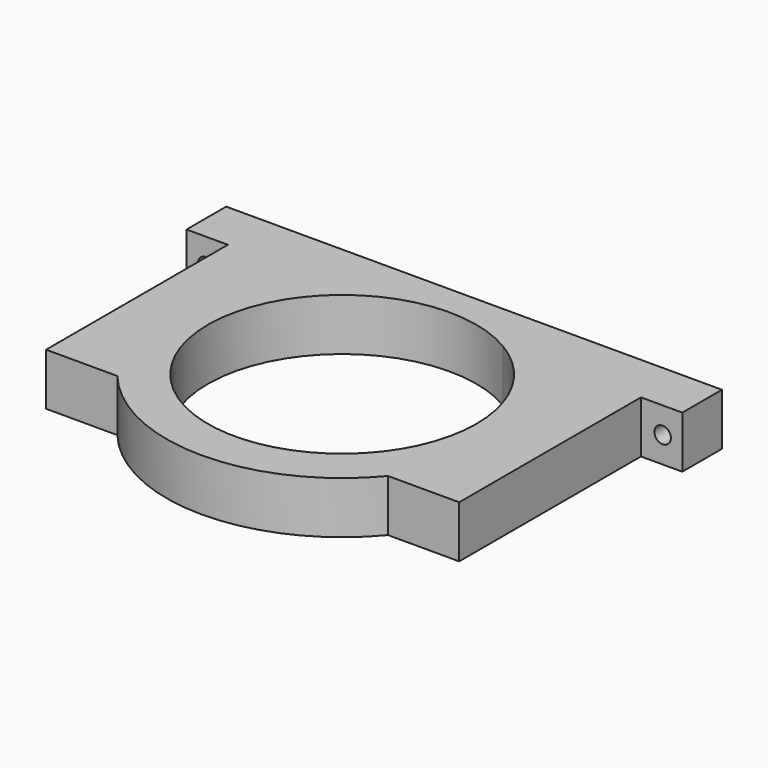
from build123d import *

# Parameters (mm, degrees)
F1_DEPTH = 12.6
F2_R     = 2
F3_DEPTH = 82.4149229208


# Not quite as in the source:
# - a feature names something its author has since deleted; it is built from what else it names


with BuildPart() as f1:
    # F0 (on Top) → F1 (new body)
    with BuildSketch(Plane.XY):
        with BuildLine():
            Line((4.3273164821, 32.1861776987), (-41.0737535205, 32.1861776987))
            Line((-41.0737535205, 32.1861776987), (-41.0737535205, 20.1861776987))
            Line((-41.0737535205, 20.1861776987), (-31.0737535205, 20.1861776987))
            Line((-31.0737535205, 20.1861776987), (-13.1215757112, 20.1861776987))
            ThreePointArc((-13.1215757112, 20.1861776987), (-5.1565247985, 27.2903947567), (4.3273164821, 32.1861776987))
        make_face()
        with BuildLine():
            Line((33.525176477, 32.1861776987), (4.3273164821, 32.1861776987))
            ThreePointArc((4.3273164821, 32.1861776987), (-5.1565247985, 27.2903947567), (-13.1215757112, 20.1861776987))
            Line((-13.1215757112, 20.1861776987), (2.2810397469, 20.1861776987))
            ThreePointArc((2.2810397469, 20.1861776987), (18.9262464795, 24.7722547779), (35.5714532121, 20.1861776987))
            Line((35.5714532121, 20.1861776987), (50.9740686703, 20.1861776987))
            ThreePointArc((50.9740686703, 20.1861776987), (43.0090177575, 27.2903947567), (33.525176477, 32.1861776987))
        make_face()
        with BuildLine():
            Line((78.9262464795, 32.1861776987), (33.525176477, 32.1861776987))
            ThreePointArc((33.525176477, 32.1861776987), (43.0090177575, 27.2903947567), (50.9740686703, 20.1861776987))
            Line((50.9740686703, 20.1861776987), (68.9262464795, 20.1861776987))
            Line((68.9262464795, 20.1861776987), (78.9262464795, 20.1861776987))
            Line((78.9262464795, 20.1861776987), (78.9262464795, 32.1861776987))
        make_face()
        with BuildLine():
            Line((68.9262464795, 20.1861776987), (50.9740686703, 20.1861776987))
            ThreePointArc((50.9740686703, 20.1861776987), (58.7275180868, 7.1755691223), (61.4262464795, -7.7277452221))
            ThreePointArc((61.4262464795, -7.7277452221), (58.9146555301, -22.121394572), (51.6767339333, -34.8138223013))
            Line((51.6767339333, -34.8138223013), (68.9262464795, -34.8138223013))
            Line((68.9262464795, -34.8138223013), (68.9262464795, 20.1861776987))
        make_face()
        with BuildLine():
            ThreePointArc((-13.8242409743, -34.8138223013), (-23.5702855343, -7.1848209158), (-13.1215757112, 20.1861776987))
            Line((-13.1215757112, 20.1861776987), (-31.0737535205, 20.1861776987))
            Line((-31.0737535205, 20.1861776987), (-31.0737535205, -34.8138223013))
            Line((-31.0737535205, -34.8138223013), (-19.9806198337, -34.8138223013))
            Line((-19.9806198337, -34.8138223013), (-13.8242409743, -34.8138223013))
        make_face()
        with BuildLine():
            Line((2.2810397469, 20.1861776987), (-13.1215757112, 20.1861776987))
            ThreePointArc((-13.1215757112, 20.1861776987), (-23.5702855343, -7.1848209158), (-13.8242409743, -34.8138223013))
            Line((-13.8242409743, -34.8138223013), (0.9653325701, -34.8138223013))
            ThreePointArc((0.9653325701, -34.8138223013), (-13.5644582908, -6.9505042503), (2.2810397469, 20.1861776987))
        make_face()
        with BuildLine():
            ThreePointArc((61.4262464795, -7.7277452221), (58.7275180868, 7.1755691223), (50.9740686703, 20.1861776987))
            Line((50.9740686703, 20.1861776987), (35.5714532121, 20.1861776987))
            ThreePointArc((35.5714532121, 20.1861776987), (47.1859281728, 8.3234351269), (51.4262464795, -7.7277452221))
            ThreePointArc((51.4262464795, -7.7277452221), (47.5617113968, -23.0985015136), (36.8871603889, -34.8138223013))
            Line((36.8871603889, -34.8138223013), (51.6767339333, -34.8138223013))
            ThreePointArc((51.6767339333, -34.8138223013), (58.9146555301, -22.121394572), (61.4262464795, -7.7277452221))
        make_face()
        with BuildLine():
            Line((0.9653325701, -34.8138223013), (-13.8242409743, -34.8138223013))
            ThreePointArc((-13.8242409743, -34.8138223013), (18.9262464795, -50.2277452221), (51.6767339333, -34.8138223013))
            Line((51.6767339333, -34.8138223013), (36.8871603889, -34.8138223013))
            ThreePointArc((36.8871603889, -34.8138223013), (18.9262464795, -40.2277452221), (0.9653325701, -34.8138223013))
        make_face()
    extrude(amount=F1_DEPTH)

    # F2 (on face) → F3 (cut, through all)
    with BuildSketch(Plane(origin=(0, 32.1861776987, 0), x_dir=(-1, 0, 0), z_dir=(0, 1, 0))):
        with Locations((-74.1762464795, 6.3)):
            Circle(F2_R)
        with Locations((36.3237535205, 6.3)):
            Circle(F2_R)
    extrude(amount=-F3_DEPTH, mode=Mode.SUBTRACT)


solid = f1.part
